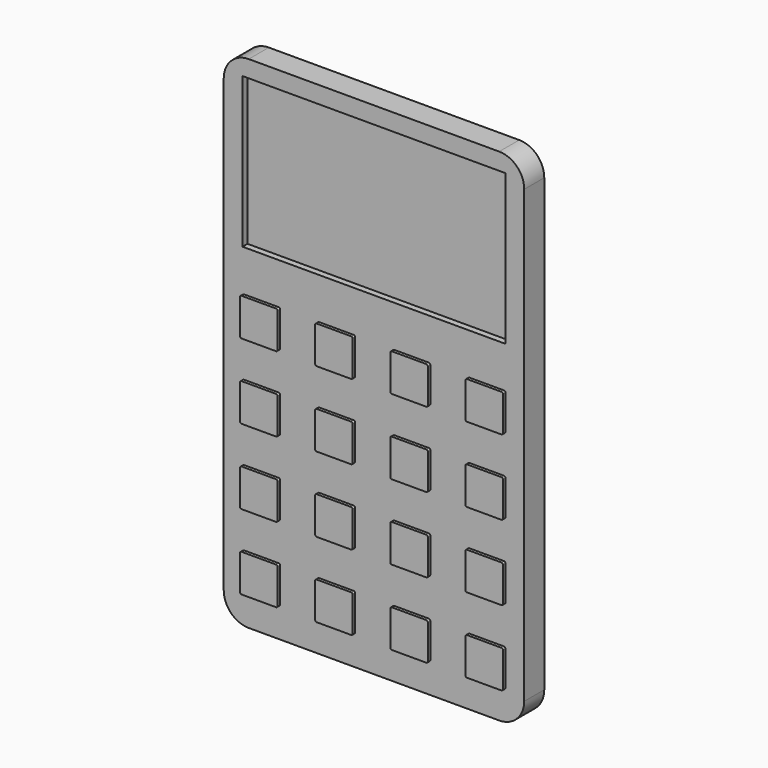
from build123d import *

# Parameters (mm, degrees)
F0_W            = 76.2
F0_H            = 127
F1_DEPTH        = 6.35
F2_W            = 66.675
F2_H            = 38.1
F3_DEPTH        = 1.5875
F4_R            = 6.35
F5_W            = 9.525
F5_H            = 9.525
F6_DEPTH        = 0.79375
F7_R            = 0.396875
F8_TEXT_SIZE    = 7.6153137747
F8_TEXT_SIZE_2  = 7.6153140981
F8_TEXT_SIZE_3  = 7.3527179969
F8_TEXT_SIZE_4  = 6.9588219048
F8_TEXT_SIZE_5  = 7.6546838197
F8_TEXT_SIZE_6  = 7.5102576779
F8_TEXT_SIZE_7  = 7.2213989269
F8_TEXT_SIZE_8  = 7.9435399837
F8_TEXT_SIZE_9  = 6.9482226132
F8_TEXT_SIZE_10 = 9.0983954983
F8_TEXT_SIZE_11 = 8.7344630932
F8_TEXT_SIZE_12 = 7.7336379844
F8_TEXT_SIZE_13 = 7.6426503559
F8_TEXT_SIZE_14 = 8.3705203401
F8_TEXT_SIZE_15 = 7.4606854469
F9_DEPTH        = 0.79375


# Not quite as in the source:
# - Text() gives the source's letters only with a copy of the font that has no kerning and outlines rounded to 1/6400 em; it was checked with that copy


with BuildPart() as f1:
    # F0 (on Front) → F1 (new body)
    with BuildSketch(Plane.XZ):
        with Locations((-16.0443431683, -1.1790953577)):
            Rectangle(F0_W, F0_H)
    extrude(amount=F1_DEPTH)

    # F2 (on face) → F3 (cut)
    with BuildSketch(Plane.XZ.offset(6.35)):
        with Locations((-16.0443431683, 38.9724979177)):
            Rectangle(F2_W, F2_H)
    extrude(amount=-F3_DEPTH, mode=Mode.SUBTRACT)

    # F4
    f4_edges = [f1.edges().sort_by_distance(p)[0] for p in [
        (-54.144343, -3.175, 62.320905),
        (22.055657, -3.175, 62.320905),
        (22.055657, -3.175, -64.679095),
        (-54.144343, -3.175, -64.679095),
    ]]
    fillet(f4_edges, radius=F4_R)

    # F5 (on face) → F6 (join)
    with BuildSketch(Plane.XZ.offset(6.35)):
        with Locations((-44.6193431683, -52.5025083224)):
            Rectangle(F5_W, F5_H)
        with Locations((-44.6193431683, -33.4525083224)):
            Rectangle(F5_W, F5_H)
        with Locations((-44.6193431683, -14.4025083224)):
            Rectangle(F5_W, F5_H)
        with Locations((-44.6193431683, 4.6474916776)):
            Rectangle(F5_W, F5_H)
        with Locations((-25.5693431683, -52.5025083224)):
            Rectangle(F5_W, F5_H)
        with Locations((-25.5693431683, -33.4525083224)):
            Rectangle(F5_W, F5_H)
        with Locations((-25.5693431683, -14.4025083224)):
            Rectangle(F5_W, F5_H)
        with Locations((-25.5693431683, 4.6474916776)):
            Rectangle(F5_W, F5_H)
        with Locations((-6.5193431683, -52.5025083224)):
            Rectangle(F5_W, F5_H)
        with Locations((-6.5193431683, -33.4525083224)):
            Rectangle(F5_W, F5_H)
        with Locations((-6.5193431683, -14.4025083224)):
            Rectangle(F5_W, F5_H)
        with Locations((-6.5193431683, 4.6474916776)):
            Rectangle(F5_W, F5_H)
        with Locations((12.5306568317, -52.5025083224)):
            Rectangle(F5_W, F5_H)
        with Locations((12.5306568317, -33.4525083224)):
            Rectangle(F5_W, F5_H)
        with Locations((12.5306568317, -14.4025083224)):
            Rectangle(F5_W, F5_H)
        with Locations((12.5306568317, 4.6474916776)):
            Rectangle(F5_W, F5_H)
    extrude(amount=F6_DEPTH)

    # F7
    f7_edges = [f1.edges().sort_by_distance(p)[0] for p in [
        (-49.381843, -6.746875, 9.409992),
        (-49.381843, -6.746875, -9.640008),
        (-49.381843, -6.746875, -28.690008),
        (-49.381843, -6.746875, -47.740008),
        (-49.381843, -6.746875, -57.265008),
        (-30.331843, -6.746875, -57.265008),
        (-30.331843, -6.746875, -38.215008),
        (-49.381843, -6.746875, -38.215008),
        (-11.281843, -6.746875, -38.215008),
        (-11.281843, -6.746875, -57.265008),
        (-11.281843, -6.746875, -19.165008),
        (-30.331843, -6.746875, -19.165008),
        (-49.381843, -6.746875, -19.165008),
        (-49.381843, -6.746875, -0.115008),
        (-39.856843, -6.746875, -0.115008),
        (-39.856843, -6.746875, -19.165008),
        (-39.856843, -6.746875, -38.215008),
        (-39.856843, -6.746875, -57.265008),
        (-39.856843, -6.746875, -47.740008),
        (-39.856843, -6.746875, -28.690008),
        (-39.856843, -6.746875, -9.640008),
        (-39.856843, -6.746875, 9.409992),
        (-20.806843, -6.746875, -47.740008),
        (-20.806843, -6.746875, -28.690008),
        (-20.806843, -6.746875, -9.640008),
        (-20.806843, -6.746875, 9.409992),
        (-1.756843, -6.746875, 9.409992),
        (17.293157, -6.746875, 9.409992),
        (-1.756843, -6.746875, -38.215008),
        (-1.756843, -6.746875, -19.165008),
        (17.293157, -6.746875, -19.165008),
        (17.293157, -6.746875, -38.215008),
        (-20.806843, -6.746875, -0.115008),
        (-20.806843, -6.746875, -19.165008),
        (-20.806843, -6.746875, -38.215008),
        (-20.806843, -6.746875, -57.265008),
        (-30.331843, -6.746875, -47.740008),
        (-30.331843, -6.746875, -28.690008),
        (-30.331843, -6.746875, -9.640008),
        (-30.331843, -6.746875, 9.409992),
        (-11.281843, -6.746875, -47.740008),
        (-1.756843, -6.746875, -57.265008),
        (-1.756843, -6.746875, -47.740008),
        (-1.756843, -6.746875, -28.690008),
        (-11.281843, -6.746875, -28.690008),
        (-11.281843, -6.746875, -9.640008),
        (-1.756843, -6.746875, -9.640008),
        (-11.281843, -6.746875, 9.409992),
        (-11.281843, -6.746875, -0.115008),
        (-1.756843, -6.746875, -0.115008),
        (7.768157, -6.746875, 9.409992),
        (7.768157, -6.746875, -0.115008),
        (17.293157, -6.746875, -0.115008),
        (17.293157, -6.746875, -9.640008),
        (7.768157, -6.746875, -9.640008),
        (7.768157, -6.746875, -19.165008),
        (-30.331843, -6.746875, -0.115008),
        (7.768157, -6.746875, -38.215008),
        (7.768157, -6.746875, -57.265008),
        (7.768157, -6.746875, -47.740008),
        (7.768157, -6.746875, -28.690008),
        (17.293157, -6.746875, -57.265008),
        (17.293157, -6.746875, -47.740008),
        (17.293157, -6.746875, -28.690008),
    ]]
    fillet(f7_edges, radius=F7_R)

    # F8 (on face) → F9 (cut)
    with BuildSketch(Plane.XZ.offset(6.35)):
        with Locations((-47.3342090845, 2.0386211108)):
            Text('7', F8_TEXT_SIZE, font='Open Sans', text_align=(TextAlign.LEFT, TextAlign.BOTTOM))
        with Locations((-28.4272246063, 1.9440860488)):
            Text('8', F8_TEXT_SIZE_2, font='Open Sans', text_align=(TextAlign.LEFT, TextAlign.BOTTOM))
        with Locations((-8.9530283585, 1.7550159246)):
            Text('9', F8_TEXT_SIZE_3, font='Open Sans', text_align=(TextAlign.LEFT, TextAlign.BOTTOM))
        with Locations((10.5211678892, 1.8495509867)):
            Text('/', F8_TEXT_SIZE_4, font='Open Sans', text_align=(TextAlign.LEFT, TextAlign.BOTTOM))
        with Locations((-47.1598468721, -17.4482930452)):
            Text('4', F8_TEXT_SIZE_5, font='Open Sans', text_align=(TextAlign.LEFT, TextAlign.BOTTOM))
        with Locations((-28.2340012491, -17.2403175384)):
            Text('5', F8_TEXT_SIZE_6, font='Open Sans', text_align=(TextAlign.LEFT, TextAlign.BOTTOM))
        with Locations((-9.3081519008, -17.1363279223)):
            Text('6', F8_TEXT_SIZE_7, font='Open Sans', text_align=(TextAlign.LEFT, TextAlign.BOTTOM))
        with Locations((9.825672023, -17.1363279223)):
            Text('*', F8_TEXT_SIZE_8, font='Open Sans', text_align=(TextAlign.LEFT, TextAlign.BOTTOM))
        with Locations((-47.6060882211, -36.1541770399)):
            Text('1', F8_TEXT_SIZE_9, font='Open Sans', text_align=(TextAlign.LEFT, TextAlign.BOTTOM))
        with Locations((-28.6401528865, -36.6143323481)):
            Text('2', F8_TEXT_SIZE_10, font='Open Sans', text_align=(TextAlign.LEFT, TextAlign.BOTTOM))
        with Locations((-9.5116868615, -36.7453508079)):
            Text('3', F8_TEXT_SIZE_11, font='Open Sans', text_align=(TextAlign.LEFT, TextAlign.BOTTOM))
        with Locations((9.6167782322, -36.0247567296)):
            Text('-', F8_TEXT_SIZE_12, font='Open Sans', text_align=(TextAlign.LEFT, TextAlign.BOTTOM))
        with Locations((-47.0560081303, -55.3766824305)):
            Text('0', F8_TEXT_SIZE_13, font='Open Sans', text_align=(TextAlign.LEFT, TextAlign.BOTTOM))
        with Locations((-28.8446582854, -55.5077008903)):
            Text('.', F8_TEXT_SIZE_14, font='Open Sans', text_align=(TextAlign.LEFT, TextAlign.BOTTOM))
        with Locations((-9.3231424689, -55.6387193501)):
            Text('(-)', F8_TEXT_SIZE_15, font='Open Sans', text_align=(TextAlign.LEFT, TextAlign.BOTTOM))
        with Locations((9.8053235561, -55.3766824305)):
            Text('=', F8_TEXT_SIZE_14, font='Open Sans', text_align=(TextAlign.LEFT, TextAlign.BOTTOM))
    extrude(amount=-F9_DEPTH, mode=Mode.SUBTRACT)


solid = f1.part
